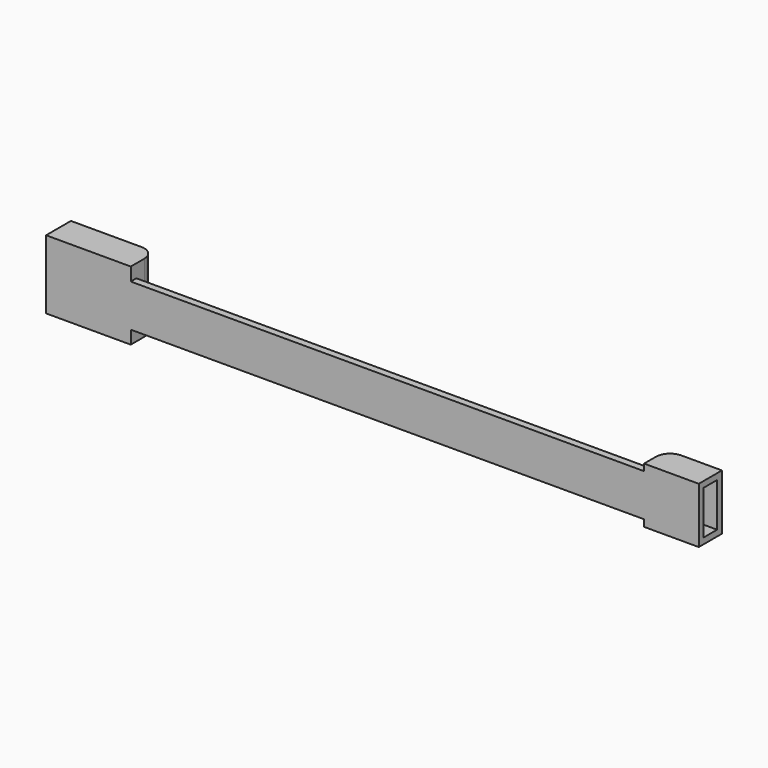
from build123d import *

# Parameters (mm, degrees)
F3_W          = 8.2
F3_H          = 15.8
F5_DEPTH      = 15.5
F4_W          = 8.8
F4_H          = 19.5
F6_DEPTH      = 24
F0_W          = 160
F0_H          = 12
F7_DEPTH      = 2
F8_W          = 4.8
F8_H          = 12.4
F9_DEPTH      = 14
F10_W         = 5.4
F10_H         = 16.1
F11_DEPTH     = 22.5
F12_TEXT_SIZE = 9.3315983476
F13_DEPTH     = 1
F14_R         = 4
F15_TEXT_SIZE = 9.7222222222
F16_DEPTH     = 1


# Not quite as in the source:
# - a feature names something its author has since deleted; it is built from what else it names
# - Text() gives the source's letters only with a copy of the font that has no kerning and outlines rounded to 1/6400 em; it was checked with that copy


with BuildPart() as f5:
    # F3 (on offset) → F5 (new body)
    with BuildSketch(Plane.YZ.offset(92.5)):
        with Locations((4.1, 6)):
            Rectangle(F3_W, F3_H)
    extrude(amount=-F5_DEPTH)



with BuildPart() as f6:
    # F4 (on offset) → F6 (new body)
    with BuildSketch(Plane.YZ.offset(-92.5)):
        with Locations((4.4, 6)):
            Rectangle(F4_W, F4_H)
    extrude(amount=F6_DEPTH)


with BuildPart() as f5_1:
    add(f5.part)

    add(f6.part)  # F7 merges F6
    # F0 (on Front) → F7 (join)
    with BuildSketch(Plane.XZ):
        with Locations((0, 6)):
            Rectangle(F0_W, F0_H)
    extrude(amount=-F7_DEPTH)

    # F8 (on offset) → F9 (cut)
    with BuildSketch(Plane.YZ.offset(92.5)):
        with Locations((4.1, 6)):
            Rectangle(F8_W, F8_H)
    extrude(amount=-F9_DEPTH, mode=Mode.SUBTRACT)

    # F10 (on offset) → F11 (cut)
    with BuildSketch(Plane.YZ.offset(-92.5)):
        with Locations((4.4, 6)):
            Rectangle(F10_W, F10_H)
    extrude(amount=F11_DEPTH, mode=Mode.SUBTRACT)

    # F12 (on face) → F13 (join)
    with BuildSketch(Plane(origin=(0, 2, 0), x_dir=(-1, 0, 0), z_dir=(0, 1, 0))):
        with Locations((-23.051964043, 2.9419420753)):
            Text('IES de Teis', F12_TEXT_SIZE, font='Open Sans', text_align=(TextAlign.LEFT, TextAlign.BOTTOM))
    extrude(amount=F13_DEPTH)

    # F14
    f14_edges = [f5_1.edges().sort_by_distance(p)[0] for p in [
        (-68.5, 8.8, 6),
        (77, 8.2, 6),
    ]]
    fillet(f14_edges, radius=F14_R)

    # F15 (on face) → F16 (join)
    with BuildSketch(Plane(origin=(0, 8.8, 0), x_dir=(-1, 0, 0), z_dir=(0, 1, 0))):
        with Locations(Location((72.4915159102, 3.2500051414), (0, 0, -0.0694432369))):
            Text('IMV', F15_TEXT_SIZE, font='Open Sans', text_align=(TextAlign.LEFT, TextAlign.BOTTOM))
    extrude(amount=F16_DEPTH)


solid = f5_1.part
